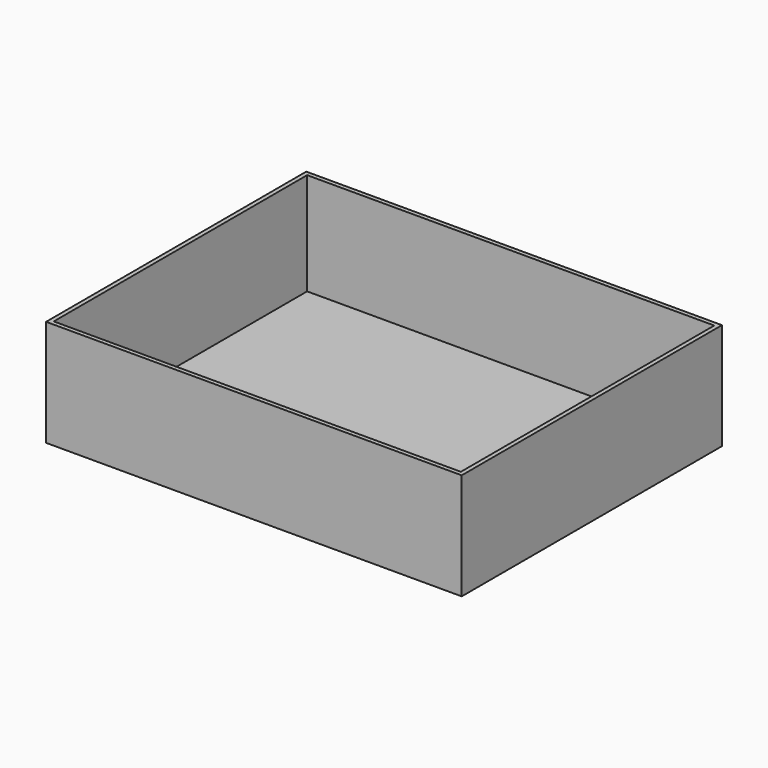
from build123d import *

# Parameters (mm, degrees)
F0_W     = 9750
F0_H     = 7630
F1_DEPTH = 2500
F2_T     = -100


# Not quite as in the source:
# - the program builds the solid bodies; features that only make, move or delete a surface that nothing else refers to are left out


with BuildPart() as f1:
    # F0 (on Top) → F1 (new body)
    with BuildSketch(Plane.XY):
        with Locations((4875, 3815)):
            Rectangle(F0_W, F0_H)
    extrude(amount=F1_DEPTH)

    # F2
    f2_openings = [f1.faces().sort_by_distance(p)[0] for p in [
        (4875, 3815, 2500),
    ]]
    offset(amount=F2_T, openings=f2_openings)


solid = f1.part
